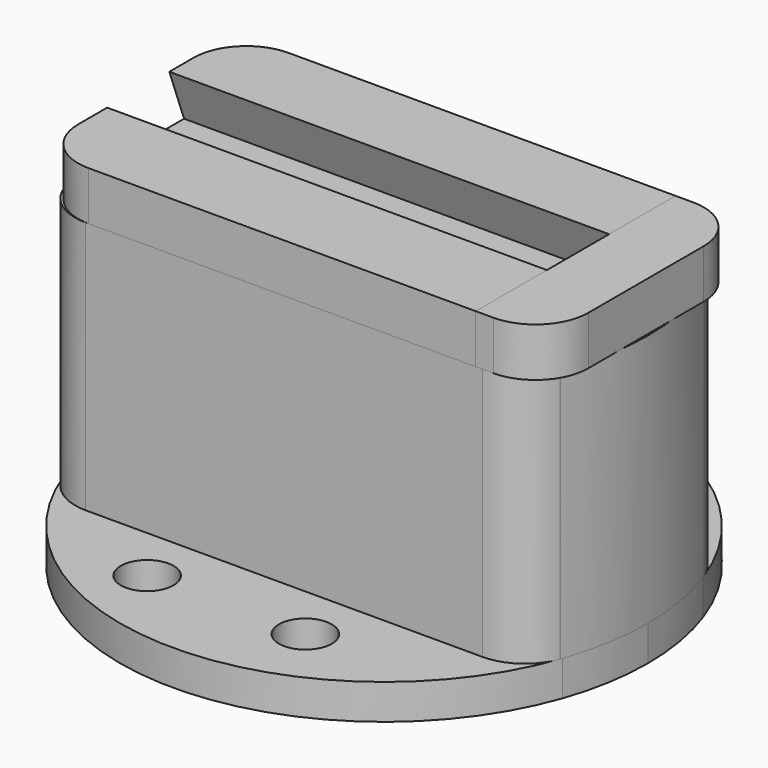
from build123d import *

# Parameters (mm, degrees)
F1_DEPTH    = 14.4
F3_DEPTH    = 2
F5_DEPTH    = 29
F6_DEPTH    = 25
F7_DEPTH    = 25
F8_T1_DEPTH = 25.219195449
F8_T3_DEPTH = 28.5421356237
F8_2_F1_R   = 3
F8_2_F2_R   = 3
F8_2_F3_R   = 3
F8_2_F4_R   = 3
F9_R        = 3
F10_R       = 4.5
F10_R_2     = 1.5
F11_DEPTH   = 2


# Not quite as in the source:
# - a fillet or chamfer that OpenCascade refuses, or shapes differently, is made with other operations: its cross-section is extruded or revolved along the edge and cut away or added
# - after a boolean that leaves OpenCascade's solid faulty, fix() repairs it


with BuildPart() as f1:
    # F0 (on Top) → F1 (new body)
    with BuildSketch(Plane.XY):
        with BuildLine():
            Line((-11.9578426148, -5.1), (-14.1063815346, -5.1))
            Line((-14.1063815346, -5.1), (-14.1063815346, -7.1))
            Line((-14.1063815346, -7.1), (-10.8899035808, -7.1))
            ThreePointArc((-10.8899035808, -7.1), (-11.4675575671, -6.123326175), (-11.9578426148, -5.1))
        make_face()
        with BuildLine():
            Line((14.1063815346, -5.1), (11.9578426148, -5.1))
            ThreePointArc((11.9578426148, -5.1), (11.4675575671, -6.123326175), (10.8899035808, -7.1))
            Line((10.8899035808, -7.1), (13.2132509247, -7.1))
            ThreePointArc((13.2132509247, -7.1), (13.6963710314, -6.1163241062), (14.1063815346, -5.1))
        make_face()
        with BuildLine():
            Line((-10.8899035808, 7.1), (-13.2132509247, 7.1))
            ThreePointArc((-13.2132509247, 7.1), (-13.6963710314, 6.1163241062), (-14.1063815346, 5.1))
            Line((-14.1063815346, 5.1), (-11.9578426148, 5.1))
            ThreePointArc((-11.9578426148, 5.1), (-11.4675575671, 6.123326175), (-10.8899035808, 7.1))
        make_face()
        with BuildLine():
            Line((13.2132509247, 7.1), (10.8899035808, 7.1))
            ThreePointArc((10.8899035808, 7.1), (11.4675575671, 6.123326175), (11.9578426148, 5.1))
            Line((11.9578426148, 5.1), (14.1063815346, 5.1))
            ThreePointArc((14.1063815346, 5.1), (13.6963710314, 6.1163241062), (13.2132509247, 7.1))
        make_face()
        with BuildLine():
            Line((11.9578426148, -5.1), (-11.9578426148, -5.1))
            ThreePointArc((-11.9578426148, -5.1), (-11.4675575671, -6.123326175), (-10.8899035808, -7.1))
            Line((-10.8899035808, -7.1), (10.8899035808, -7.1))
            ThreePointArc((10.8899035808, -7.1), (11.4675575671, -6.123326175), (11.9578426148, -5.1))
        make_face()
        with BuildLine():
            Line((14.1063815346, 5.1), (11.9578426148, 5.1))
            ThreePointArc((11.9578426148, 5.1), (13, 0), (11.9578426148, -5.1))
            Line((11.9578426148, -5.1), (14.1063815346, -5.1))
            ThreePointArc((14.1063815346, -5.1), (15, 0), (14.1063815346, 5.1))
        make_face()
        with BuildLine():
            Line((10.8899035808, 7.1), (-10.8899035808, 7.1))
            ThreePointArc((-10.8899035808, 7.1), (-11.4675575671, 6.123326175), (-11.9578426148, 5.1))
            Line((-11.9578426148, 5.1), (11.9578426148, 5.1))
            ThreePointArc((11.9578426148, 5.1), (11.4675575671, 6.123326175), (10.8899035808, 7.1))
        make_face()
    extrude(amount=F1_DEPTH)

    # F8: fillet of radius 3 on 4 edges, made by hand

    # F8_s2 → F8_t1 (cut)
    with BuildSketch(Plane.XY.offset(-5.4095977245)):
        with BuildLine():
            ThreePointArc((14.0973180073, 5.125), (12.9990458537, 6.5571324751), (11.2778544059, 7.1))
            Line((11.2778544059, 7.1), (13.2132509247, 7.1))
            ThreePointArc((13.2132509247, 7.1), (13.6909440908, 6.1284622787), (14.0973180073, 5.125))
        make_face()
        with BuildLine():
            ThreePointArc((11.2778544059, -7.1), (12.9990458537, -6.5571324751), (14.0973180073, -5.125))
            ThreePointArc((14.0973180073, -5.125), (13.6909440908, -6.1284622787), (13.2132509247, -7.1))
            Line((13.2132509247, -7.1), (11.2778544059, -7.1))
        make_face()
        with BuildLine():
            ThreePointArc((-11.2778544059, 7.1), (-12.9990458537, 6.5571324751), (-14.0973180073, 5.125))
            ThreePointArc((-14.0973180073, 5.125), (-13.6909440908, 6.1284622787), (-13.2132509247, 7.1))
            Line((-13.2132509247, 7.1), (-11.2778544059, 7.1))
        make_face()
    extrude(amount=F8_T1_DEPTH, mode=Mode.SUBTRACT)

    # F8_s4 → F8_t3 (cut)
    with BuildSketch(Plane.XY.offset(-7.0710678119)):
        with BuildLine():
            ThreePointArc((-14.1063815346, -5.1), (-13.0100052174, -6.5494897428), (-11.2779544099, -7.1))
            Line((-11.2779544099, -7.1), (-14.1063815346, -7.1))
            Line((-14.1063815346, -7.1), (-14.1063815346, -5.1))
        make_face()
    extrude(amount=F8_T3_DEPTH, mode=Mode.SUBTRACT)

    # F10 (on Top) → F11 (join)
    with BuildSketch(Plane.XY):
        with BuildLine():
            ThreePointArc((14.1452126344, -4.9912883635), (14.7847588671, -2.5319765485), (15, 0))
            ThreePointArc((15, 0), (14.7831963499, 2.5410835644), (14.1390525758, 5.0087116365))
            Line((14.1390525758, 5.0087116365), (-14.1390525758, 5.0087116365))
            ThreePointArc((-14.1390525758, 5.0087116365), (-14.999997154, 0.0092400861), (-14.1452126344, -4.9912883635))
            Line((-14.1452126344, -4.9912883635), (14.1452126344, -4.9912883635))
        make_face()
        with Locations((0.0035419917, 0.0087116365)):
            Circle(F10_R, mode=Mode.SUBTRACT)
        with BuildLine():
            Line((-14.1390525758, 5.0087116365), (14.1390525758, 5.0087116365))
            ThreePointArc((14.1390525758, 5.0087116365), (0, 15), (-14.1390525758, 5.0087116365))
        make_face()
        with Locations((-7.1710880957, 8.6605090521)):
            Circle(F10_R_2, mode=Mode.SUBTRACT)
        with Locations((5.7189119043, 8.6543741425)):
            Circle(F10_R_2, mode=Mode.SUBTRACT)
        with BuildLine():
            ThreePointArc((-14.1452126344, -4.9912883635), (0, -15), (14.1452126344, -4.9912883635))
            Line((14.1452126344, -4.9912883635), (-14.1452126344, -4.9912883635))
        make_face()
        with Locations((-5.2289596802, -10.2956258575)):
            Circle(F10_R_2, mode=Mode.SUBTRACT)
        with Locations((3.7661575137, -10.2956258575)):
            Circle(F10_R_2, mode=Mode.SUBTRACT)
    extrude(amount=-F11_DEPTH)

    add(f1.part.fix(), mode=Mode.REPLACE)


with BuildPart() as f3:
    # F2 (on face) → F3 (new body)
    with BuildSketch(Plane.XY.offset(14.4)):
        with BuildLine():
            Line((-14.1063815346, 5.1), (-14.1063815346, -5.1))
            Line((-14.1063815346, -5.1), (11.9578426148, -5.1))
            ThreePointArc((11.9578426148, -5.1), (13, 0), (11.9578426148, 5.1))
            Line((11.9578426148, 5.1), (-14.1063815346, 5.1))
        make_face()
    extrude(amount=-F3_DEPTH)


with BuildPart() as f5:
    # F4 (on face) → F5 (new body)
    with BuildSketch(Plane(origin=(-14.1063815346, 0, 0), x_dir=(0, -1, 0), z_dir=(-1, 0, 0))):
        Polygon((5.1, 14.4), (5.4331574369, 14.4), (7.1, 14.4), (7.1, 17.1767032981), (2.039092524, 17.1767032981), (3.2555045802, 14.4), align=None)
        Polygon((-4.7668425631, 14.4), (-3.4248761367, 14.4), (-2.377835637, 17.1767032981), (-7.1, 17.1767032981), (-7.1, 14.4), (-5.1, 14.4), align=None)
        Polygon((-3.4248761367, 14.4), (3.2555045802, 14.4), (2.039092524, 17.1767032981), (-2.377835637, 17.1767032981), align=None)
    extrude(amount=-F5_DEPTH)


with BuildPart() as f6:
    # F4 (on face) → F6 (new body)
    with BuildSketch(Plane(origin=(-14.1063815346, 0, 0), x_dir=(0, -1, 0), z_dir=(-1, 0, 0))):
        Polygon((3.2555045802, 14.4), (5.4331574369, 14.4), (7.1, 14.4), (7.1, 17.1767032981), (2.039092524, 17.1767032981), align=None)
        Polygon((-3.4248761367, 14.4), (3.2555045802, 14.4), (2.039092524, 17.1767032981), (-2.377835637, 17.1767032981), align=None)
        Polygon((-4.7668425631, 14.4), (-3.4248761367, 14.4), (-2.377835637, 17.1767032981), (-7.1, 17.1767032981), (-7.1, 14.4), align=None)
    extrude(amount=-F6_DEPTH)


with BuildPart() as f7_tool:
    # F4 (on face) → F7 (new body)
    with BuildSketch(Plane(origin=(-14.1063815346, 0, 0), x_dir=(0, -1, 0), z_dir=(-1, 0, 0))):
        Polygon((-3.4248761367, 14.4), (3.2555045802, 14.4), (2.039092524, 17.1767032981), (-2.377835637, 17.1767032981), align=None)
    extrude(amount=-F7_DEPTH)


with BuildPart() as f5_1:
    add(f5.part)

    # F7: cut by f7_tool
    add(f7_tool.part, mode=Mode.SUBTRACT)

    # F8#2: fillet of radius 3 on 4 edges, made by hand

    # F8_2_f1
    f8_2_f1_edges = [f5_1.edges().sort_by_distance(p)[0] for p in [
        (-14.1063815346, -7.1, 15.788351649),
    ]]
    fillet(f8_2_f1_edges, radius=F8_2_F1_R)

    # F8_2_f2
    f8_2_f2_edges = [f5_1.edges().sort_by_distance(p)[0] for p in [
        (14.8936184654, -7.1, 15.788351649),
    ]]
    fillet(f8_2_f2_edges, radius=F8_2_F2_R)

    # F8_2_f3
    f8_2_f3_edges = [f5_1.edges().sort_by_distance(p)[0] for p in [
        (14.8936184654, 7.1, 15.788351649),
    ]]
    fillet(f8_2_f3_edges, radius=F8_2_F3_R)

    # F8_2_f4
    f8_2_f4_edges = [f5_1.edges().sort_by_distance(p)[0] for p in [
        (-14.1063815346, 7.1, 15.788351649),
    ]]
    fillet(f8_2_f4_edges, radius=F8_2_F4_R)


with BuildPart() as f6_1:
    add(f6.part)

    # F7: cut by f7_tool
    add(f7_tool.part, mode=Mode.SUBTRACT)

    # F9
    f9_edges = [f6_1.edges().sort_by_distance(p)[0] for p in [
        (-14.106382, 7.1, 15.788352),
        (-14.106382, -7.1, 15.788352),
    ]]
    fillet(f9_edges, radius=F9_R)


solid = Compound([f1.part, f3.part, f5_1.part, f6_1.part])
